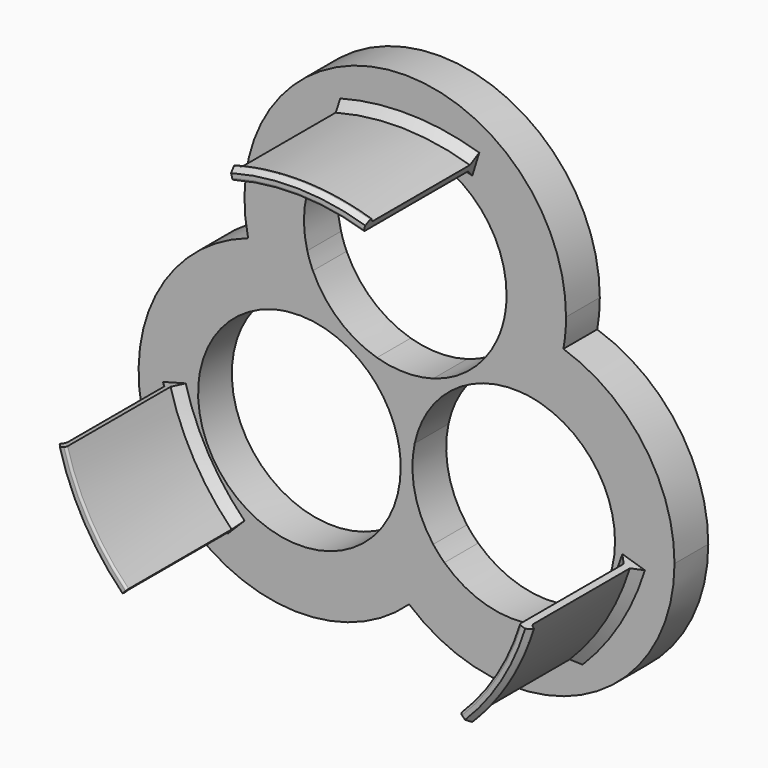
from build123d import *

# Parameters (mm, degrees)
F1_DEPTH = 1
F5_DEPTH = 25.4
F6_SIZE  = 0.2032
F7_R     = 0.0254


with BuildPart() as f1:
    # F0 (on Front) → F1 (new body)
    with BuildSketch(Plane.XZ):
        with BuildLine():
            ThreePointArc((-3.1719905538, 0.8104133692), (-2.9789481059, 0.8573735562), (-2.7826833559, 0.8882085007))
            ThreePointArc((-2.7826833559, 0.8882085007), (-2.54, 1.4424427198), (-2.1883394383, 1.9347897826))
            ThreePointArc((-2.1883394383, 1.9347897826), (-2.2624018983, 2.119141072), (-2.3209650279, 2.3089857605))
            ThreePointArc((-2.3209650279, 2.3089857605), (-3.0314381709, 2.2775636636), (-3.7236948272, 2.1146521631))
            ThreePointArc((-3.7236948272, 2.1146521631), (-3.5089712063, 1.4366748761), (-3.1719905538, 0.8104133692))
        make_face()
        with BuildLine():
            ThreePointArc((-2.7826833559, 0.8882085007), (-1.7552661043, 0.7826291226), (-0.8673282268, 0.2550880913))
            ThreePointArc((-0.8673282268, 0.2550880913), (-0.7736155948, 0.4382816345), (-0.6701492774, 0.616148587))
            ThreePointArc((-0.6701492774, 0.616148587), (-1.5739895442, 1.10881982), (-2.1883394383, 1.9347897826))
            ThreePointArc((-2.1883394383, 1.9347897826), (-2.54, 1.4424427198), (-2.7826833559, 0.8882085007))
        make_face()
        with BuildLine():
            ThreePointArc((0.0915085685, -4.2812712036), (-0.4030364452, -3.7702089133), (-0.7939885782, -3.1761416908))
            ThreePointArc((-0.7939885782, -3.1761416908), (-4.5700075585, -2.7260345936), (-3.1719905538, 0.8104133692))
            ThreePointArc((-3.1719905538, 0.8104133692), (-3.5089712063, 1.4366748761), (-3.7236948272, 2.1146521631))
            ThreePointArc((-3.7236948272, 2.1146521631), (-5.7806778186, -3.4482060491), (0.0915085685, -4.2812712036))
        make_face()
        with BuildLine():
            ThreePointArc((0.6627274406, -2.8448257134), (0.0624196597, -2.9203329923), (-0.5405661999, -2.8705451022))
            ThreePointArc((-0.5405661999, -2.8705451022), (-0.6609484293, -3.028591819), (-0.7939885782, -3.1761416908))
            ThreePointArc((-0.7939885782, -3.1761416908), (-0.4030364452, -3.7702089133), (0.0915085685, -4.2812712036))
            ThreePointArc((0.0915085685, -4.2812712036), (0.5637648419, -3.7495443495), (0.9289761445, -3.1393147701))
            ThreePointArc((0.9289761445, -3.1393147701), (0.7897528718, -2.9975842997), (0.6627274406, -2.8448257134))
        make_face()
        with BuildLine():
            ThreePointArc((0.9289761445, -3.1393147701), (0.5637648419, -3.7495443495), (0.0915085685, -4.2812712036))
            ThreePointArc((0.0915085685, -4.2812712036), (4.1627448452, -4.8490549435), (6.3802439522, -1.3878353744))
            ThreePointArc((6.3802439522, -1.3878353744), (5.6526747439, 0.8515217687), (3.7478447845, 2.235609986))
            ThreePointArc((3.7478447845, 2.235609986), (3.5557756025, 1.5525849076), (3.2403932296, 0.9170160386))
            ThreePointArc((3.2403932296, 0.9170160386), (4.4898792562, 0.0531505345), (4.9705439522, -1.3878353744))
            ThreePointArc((4.9705439522, -1.3878353744), (3.5246822611, -3.590217631), (0.9289761445, -3.1393147701))
        make_face()
        with BuildLine():
            ThreePointArc((-0.1876310066, -0.8843770648), (-0.1282124051, -1.1878238615), (-0.1082960345, -1.4963913043))
            ThreePointArc((-0.1082960345, -1.4963913043), (-0.2189124208, -2.2166614196), (-0.5405661999, -2.8705451022))
            ThreePointArc((-0.5405661999, -2.8705451022), (0.0624196597, -2.9203329923), (0.6627274406, -2.8448257134))
            ThreePointArc((0.6627274406, -2.8448257134), (0.2278326149, -1.9118098174), (0.2237573797, -0.8824238043))
            ThreePointArc((0.2237573797, -0.8824238043), (0.0180895692, -0.8889570559), (-0.1876310066, -0.8843770648))
        make_face()
        with BuildLine():
            ThreePointArc((-0.8673282268, 0.2550880913), (-0.4471845105, -0.2667480151), (-0.1876310066, -0.8843770648))
            ThreePointArc((-0.1876310066, -0.8843770648), (0.0180895692, -0.8889570559), (0.2237573797, -0.8824238043))
            ThreePointArc((0.2237573797, -0.8824238043), (0.4565057727, -0.2504915396), (0.8556364959, 0.2919150121))
            ThreePointArc((0.8556364959, 0.2919150121), (0.7634857496, 0.4554234405), (0.6633945194, 0.6141953265))
            ThreePointArc((0.6633945194, 0.6141953265), (-0.0035157497, 0.5207025748), (-0.6701492774, 0.616148587))
            ThreePointArc((-0.6701492774, 0.616148587), (-0.7736155948, 0.4382816345), (-0.8673282268, 0.2550880913))
        make_face()
        with BuildLine():
            ThreePointArc((2.1883394383, 1.9347897826), (2.5085960345, 1.4963913043), (2.7421898737, 1.0062980158))
            ThreePointArc((2.7421898737, 1.0062980158), (2.9936514378, 0.9748254542), (3.2403932296, 0.9170160386))
            ThreePointArc((3.2403932296, 0.9170160386), (3.5557756025, 1.5525849076), (3.7478447845, 2.235609986))
            ThreePointArc((3.7478447845, 2.235609986), (3.0555813535, 2.3911258065), (2.3464865725, 2.4155884299))
            ThreePointArc((2.3464865725, 2.4155884299), (2.2801213941, 2.1710089879), (2.1883394383, 1.9347897826))
        make_face()
        with BuildLine():
            ThreePointArc((0.6633945194, 0.6141953265), (0.7634857496, 0.4554234405), (0.8556364959, 0.2919150121))
            ThreePointArc((0.8556364959, 0.2919150121), (1.7202222338, 0.8569147606), (2.7421898737, 1.0062980158))
            ThreePointArc((2.7421898737, 1.0062980158), (2.5085960345, 1.4963913043), (2.1883394383, 1.9347897826))
            ThreePointArc((2.1883394383, 1.9347897826), (1.5713335326, 1.1065163216), (0.6633945194, 0.6141953265))
        make_face()
        with BuildLine():
            ThreePointArc((3.81, 2.921), (-0.4054767, 6.7093622643), (-3.7236948272, 2.1146521631))
            ThreePointArc((-3.7236948272, 2.1146521631), (-3.0314381709, 2.2775636636), (-2.3209650279, 2.3089857605))
            ThreePointArc((-2.3209650279, 2.3089857605), (-0.3085674429, 5.3013836294), (2.4003, 2.921))
            ThreePointArc((2.4003, 2.921), (2.3868087282, 2.6668658129), (2.3464865725, 2.4155884299))
            ThreePointArc((2.3464865725, 2.4155884299), (3.0555813535, 2.3911258065), (3.7478447845, 2.235609986))
            ThreePointArc((3.7478447845, 2.235609986), (3.7944293793, 2.5768987278), (3.81, 2.921))
        make_face()
    extrude(amount=-F1_DEPTH)

    # F2 (on Right) → F3 (revolve)
    with BuildSketch(Plane.YZ):
        with BuildLine():
            Line((-3.2512, 5.588), (0, 5.588))
            Line((0, 5.588), (0, 5.7404))
            Line((0, 5.7404), (-3.048, 5.7404))
            ThreePointArc((-3.048, 5.7404), (-3.119842049, 5.770157951), (-3.1496, 5.842))
            Line((-3.1496, 5.842), (-3.1496, 5.8674))
            Line((-3.1496, 5.8674), (-3.302, 5.7395212162))
            Line((-3.302, 5.7395212162), (-3.302, 5.6388))
            ThreePointArc((-3.302, 5.6388), (-3.2871210245, 5.6028789755), (-3.2512, 5.588))
        make_face()
    revolve(axis=Axis((0, -1.6292430228, 0), (0, -1, 0)))

    # F4 (on face) → F5 (cut)
    with BuildSketch(Plane.XZ):
        Polygon((-3.2870018728, 12.2672579939), (-12.2672579939, -3.2870018728), (0, 0), align=None)
        Polygon((3.7478447845, 12.1343998398), (0, 0), (12.1343998398, -3.7478447845), align=None)
        Polygon((8.9802561211, -8.9802561211), (0, 0), (-8.9802561211, -8.9802561211), align=None)
    extrude(amount=F5_DEPTH, mode=Mode.SUBTRACT)

    # F6
    f6_edges = [f1.edges().sort_by_distance(p)[0] for p in [
        (4.91625, 0, -2.963559),
        (4.78573, 0, -2.88488),
        (-4.971332, 0, -2.8702),
        (-4.83935, 0, -2.794),
        (0.108392, 0, 5.739377),
        (0.105515, 0, 5.587004),
    ]]
    chamfer(f6_edges, length=F6_SIZE)

    # F7
    f7_edges = [f1.edges().sort_by_distance(p)[0] for p in [
        (0.11079, -3.1496, 5.866354),
        (-5.081317, -3.1496, -2.9337),
        (5.025016, -3.1496, -3.029124),
    ]]
    fillet(f7_edges, radius=F7_R)


solid = f1.part
